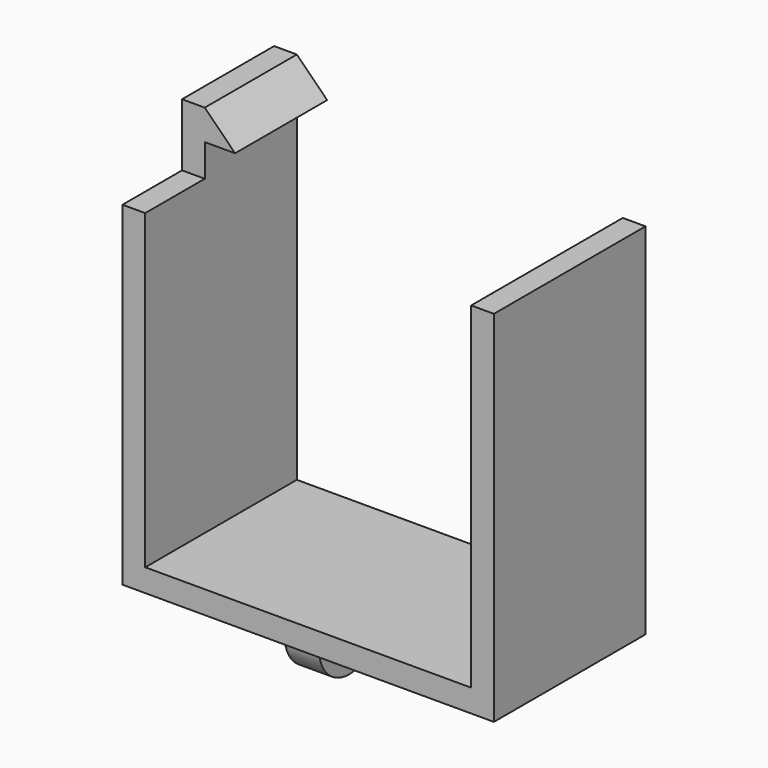
from build123d import *

# Parameters (mm, degrees)
F0_W     = 43
F0_H     = 3
F1_DEPTH = 25
F2_W     = 4.5
F2_H     = 10
F3_DEPTH = 14
F4_R     = 4.99999
F6_DEPTH = 5
F7_W     = 9.8148105666
F7_H     = 8.2614529669
F8_DEPTH = 7


# Not quite as in the source:
# - a fillet or chamfer is up to 0.001 mm smaller than in the source, because OpenCascade refuses the exact size


with BuildPart() as f1:
    # F0 (on Front) → F1 (new body)
    with BuildSketch(Plane.XZ):
        Polygon((0, 52.4), (0, 48.4), (4, 48.4), align=None)
        Polygon((-3, 0), (0, 0), (0, 3), (0, 48.4), (0, 52.4), (-3, 52.4), align=None)
        with Locations((21.5, 1.5)):
            Rectangle(F0_W, F0_H)
        Polygon((43, 3), (43, 0), (46, 0), (46, 47.4), (43, 47.4), align=None)
    extrude(amount=F1_DEPTH)

    # F2 (on face) → F3 (join)
    with BuildSketch(Plane(origin=(0, 0, 0), x_dir=(1, 0, 0), z_dir=(0, 0, -1))):
        with Locations((8.6824605241, 5.0298511051)):
            Rectangle(F2_W, F2_H)
    extrude(amount=F3_DEPTH)

    # F4 (radius 5 in the source; OpenCascade refuses exactly that, so slightly less here)
    f4_edges = [f1.edges().sort_by_distance(p)[0] for p in [
        (8.682461, -10.029851, -14),
        (8.682461, -0.029851, -14),
    ]]
    fillet(f4_edges, radius=F4_R)

    # F5 (on face) → F6 (cut)
    with BuildSketch(Plane(origin=(6.4324605241, 0, 0), x_dir=(0, -1, 0), z_dir=(-1, 0, 0))):
        with BuildLine():
            ThreePointArc((5.0298511051, -7.45), (3.9338580131, -10.0959613868), (6.5798194, -8.9999682949))
            ThreePointArc((6.5798194, -8.9999682949), (6.125844197, -7.9039752029), (5.0298511051, -7.45))
        make_face()
    extrude(amount=-F6_DEPTH, mode=Mode.SUBTRACT)

    # F7 (on face) → F8 (cut)
    with BuildSketch(Plane(origin=(-3, 0, 0), x_dir=(0, -1, 0), z_dir=(-1, 0, 0))):
        with Locations((20.0925947167, 48.2692735165)):
            Rectangle(F7_W, F7_H)
    extrude(amount=-F8_DEPTH, mode=Mode.SUBTRACT)


solid = f1.part
